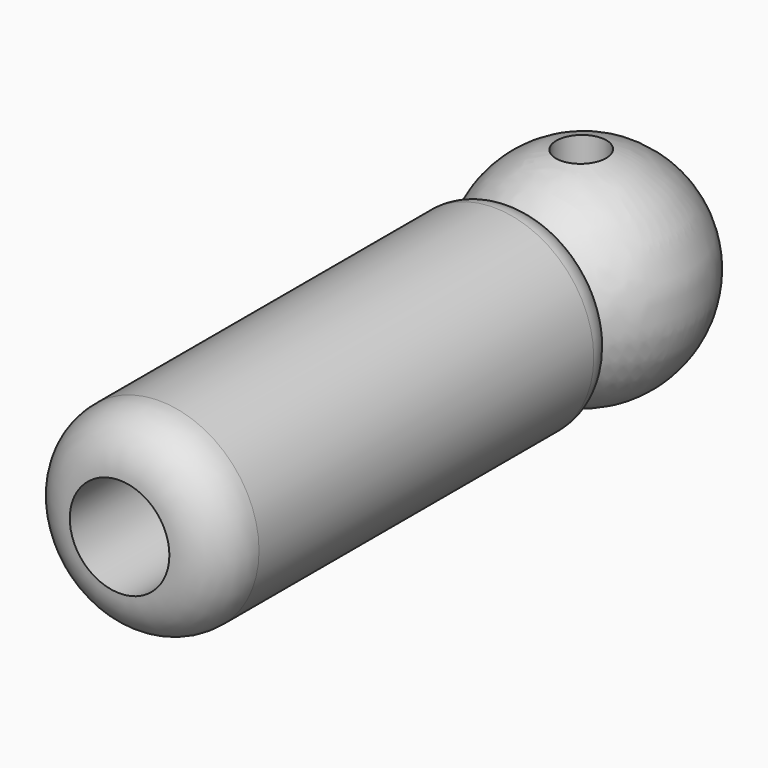
from build123d import *

# Parameters (mm, degrees)
F6_R     = 12.7
F0_DEPTH = 63.5
F1_R     = 6.35
F2_R     = 3.81
F5_D     = 6.35
F5_DEPTH = 13.8140768323
F7_D     = 6.35
F8_DEPTH = 60.325


with BuildPart() as f0:
    # F6 (on Front) → F0 (new body)
    with BuildSketch(Plane.XZ):
        Circle(F6_R)
    extrude(amount=F0_DEPTH)

    # F1
    f1_edges = [f0.edges().sort_by_distance(p)[0] for p in [
        (-12.7, -63.5, 0),
    ]]
    fillet(f1_edges, radius=F1_R)

    # F2
    f2_edges = [f0.edges().sort_by_distance(p)[0] for p in [
        (-12.7, 0, 0),
    ]]
    fillet(f2_edges, radius=F2_R)

    # F3 (on Top) → F4 (revolve)
    with BuildSketch(Plane.XY):
        with BuildLine():
            Line((0.0938863529, 0), (9.398, 0))
            ThreePointArc((9.398, 0), (12.9224991184, 15.3285868193), (3.58e-06, 24.2950118021))
            Line((3.58e-06, 24.2950118021), (0.0938863529, 0))
        make_face()
    revolve(axis=Axis((0.0470116362, 12.1302530893, 0), (-0.003864253, 0.9999925337, 0)))

    # F5 (through all, one way)
    with BuildSketch(Plane.XY):
        with Locations((-0.1612169292, 10.2674360951)):
            Circle(F5_D / 2)
    extrude(amount=-F5_DEPTH, mode=Mode.SUBTRACT)

    # F7 (through all)
    with Locations(Plane(origin=(0, 0, 0), x_dir=(1, 0, 0), z_dir=(0, 0, -1))):
        with Locations((-0.1612169292, -10.2674360951)):
            Hole(F7_D / 2)

    # F8 (cut): a face of the model
    f8_faces = [f0.faces().sort_by_distance(p)[0] for p in [
        (0, -63.5, 0),
    ]]
    extrude(f8_faces, amount=-F8_DEPTH, mode=Mode.SUBTRACT)


solid = f0.part
